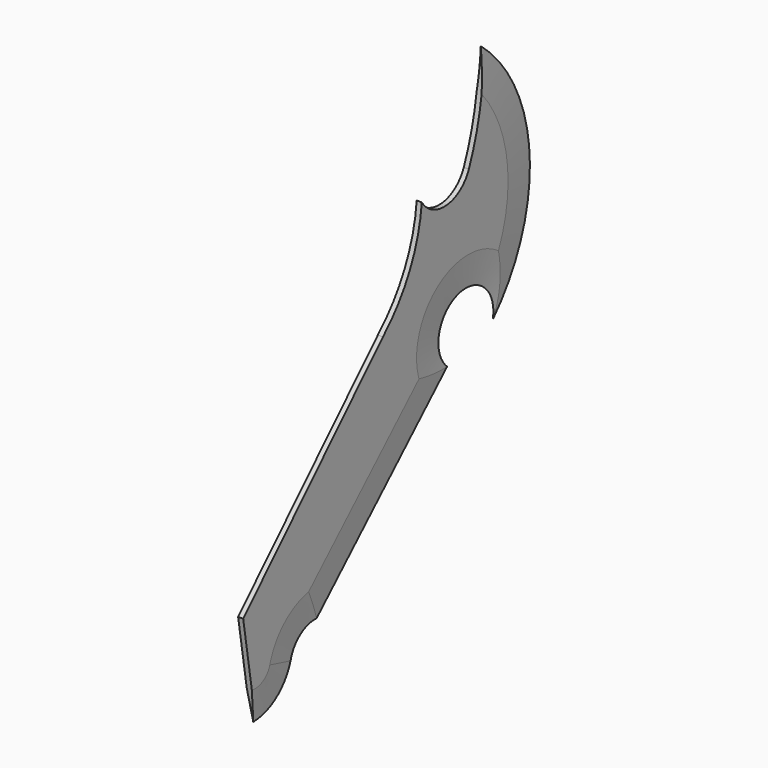
from build123d import *

# Parameters (mm, degrees)
F1_DEPTH = 0.254
F2_SIZE2 = 0.254
F2_SIZE  = 3.048
F3_SIZE2 = 0.25399
F3_SIZE  = 3.04799


# Not quite as in the source:
# - a fillet or chamfer is up to 0.001 mm smaller than in the source, because OpenCascade refuses the exact size


with BuildPart() as f1:
    # F0 (on Right) → F1 (new body, symmetric)
    with BuildSketch(Plane.YZ):
        with BuildLine():
            ThreePointArc((-9.1647058725, -19.4605849683), (-7.9769017154, -17.6542353956), (-5.9044379741, -17.0388724655))
            Line((-5.9044379741, -17.0388724655), (10.4197403416, -1.4963007998))
            ThreePointArc((10.4197403416, -1.4963007998), (11.7207158788, 4.2992743145), (16.1321125925, 0.321736472))
            ThreePointArc((16.1321125925, 0.321736472), (20.7425449922, 12.9991270925), (14.6297309548, 25.024343282))
            ThreePointArc((14.6297309548, 25.024343282), (14.2521620564, 19.9192816811), (12.8257451579, 15.0030283257))
            ThreePointArc((12.8257451579, 15.0030283257), (10.0409395244, 12.9549949897), (6.9327647798, 14.4678838551))
            ThreePointArc((6.9327647798, 14.4678838551), (5.4294099174, 9.0746087463), (2.0746421069, 4.5920843259))
            Line((2.0746421069, 4.5920843259), (-15.4057918116, -13.1268743426))
            Line((-15.4057918116, -13.1268743426), (-13.8271413743, -22.945875302))
            ThreePointArc((-13.8271413743, -22.945875302), (-10.9300822918, -21.9601824865), (-9.1647058725, -19.4605849683))
        make_face()
    extrude(amount=F1_DEPTH, both=True)

    # F2
    f2_edges = [f1.edges().sort_by_distance(p)[0] for p in [
        (-0.254, -7.976902, -17.654235),
        (-0.254, -10.930082, -21.960182),
        (-0.254, 2.257651, -9.267587),
        (-0.254, 11.720716, 4.299274),
        (-0.254, 20.742545, 12.999127),
    ]]
    f2_side = f1.faces().sort_by_distance((-0.254, 3.800981, -0.184421))[0]
    chamfer(f2_edges, length=F2_SIZE, length2=F2_SIZE2, reference=f2_side)

    # F3 (size 3.048 and 0.254 in the source; OpenCascade refuses exactly that, so slightly less here)
    f3_edges = [f1.edges().sort_by_distance(p)[0] for p in [
        (0.254, 20.742545, 12.999127),
        (0.254, 11.720716, 4.299274),
        (0.254, 2.257651, -9.267587),
        (0.254, -7.976902, -17.654235),
        (0.254, -10.930082, -21.960182),
    ]]
    f3_side = f1.faces().sort_by_distance((0.254, 3.800981, -0.184421))[0]
    chamfer(f3_edges, length=F3_SIZE, length2=F3_SIZE2, reference=f3_side)


solid = f1.part
